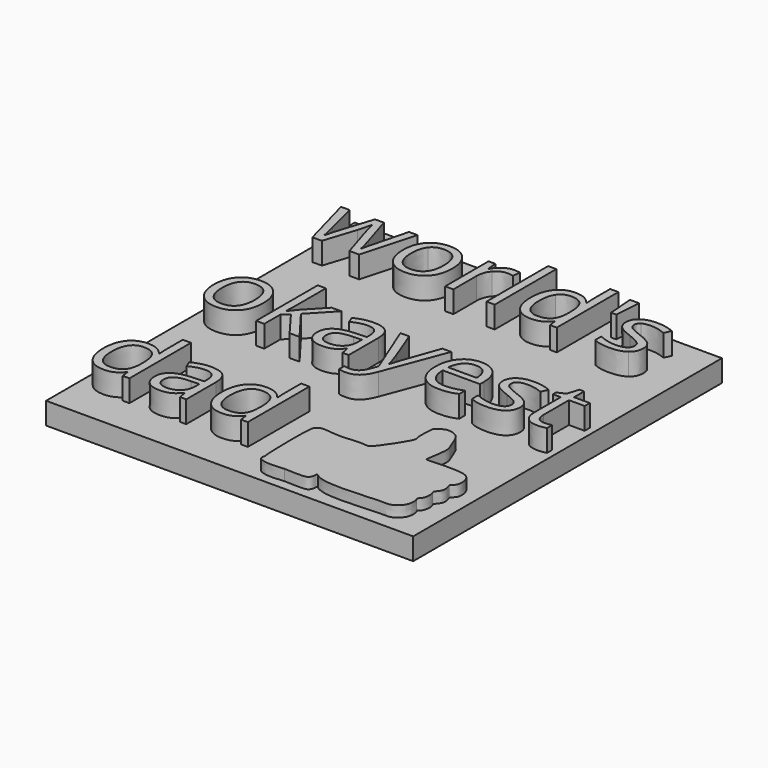
from build123d import *

# Parameters (mm, degrees)
F0_W         = 0.954216132
F0_H         = 0.4688345157
F0_H_2       = 8.4721154837
F1_DEPTH     = 5.08
F0_TEXT_SIZE = 11.7668270607
F2_DEPTH     = 5.08
F3_DEPTH     = 5.08
F4_DEPTH     = 2.54
F6_DEPTH     = 1.27


# Not quite as in the source:
# - Text() gives the source's letters only with a copy of the font that has no kerning and outlines rounded to 1/6400 em; it was checked with that copy


with BuildPart() as f1:
    # F0 (on Top) → F1 (new body)
    with BuildSketch(Plane.XY):
        with Locations((1.2318397079, 22.6472947877)):
            Rectangle(F0_W, F0_H)
        with Locations((8.4426984161, 22.6472947877)):
            Rectangle(F0_W, F0_H)
        with Locations((1.2318397079, 18.176819788)):
            Rectangle(F0_W, F0_H_2)
        with BuildLine():
            Line((8.9198064821, 22.4128775299), (7.9655903501, 22.4128775299))
            Line((7.9655903501, 22.4128775299), (7.9655903501, 20.3187500264))
            Line((7.9655903501, 20.3187500264), (7.9894917176, 19.8756554449))
            Line((7.9894917176, 19.8756554449), (8.0299401856, 19.421529463))
            Line((8.0299401856, 19.421529463), (7.9545589497, 19.421529463))
            add(Edge.make_bspline(
                [(5.9891311172, 20.3536827942), (7.2706121268, 20.3536827942), (7.9545589497, 19.421529463)],
                knots=[0, 0, 0, 1, 1, 1], degree=2))
            add(Edge.make_bspline(
                [(4.069667453, 19.4913949987), (4.759129976, 20.3536827942), (5.9891311172, 20.3536827942)],
                knots=[0, 0, 0, 1, 1, 1], degree=2))
            add(Edge.make_bspline(
                [(3.3802049299, 17.0718411843), (3.3802049299, 18.6291072031), (4.069667453, 19.4913949987)],
                knots=[0, 0, 0, 1, 1, 1], degree=2))
            add(Edge.make_bspline(
                [(4.0669096029, 14.6697537539), (3.3802049299, 15.5145751655), (3.3802049299, 17.0718411843)],
                knots=[0, 0, 0, 1, 1, 1], degree=2))
            add(Edge.make_bspline(
                [(5.9891311172, 13.8249323423), (4.7536142759, 13.8249323423), (4.0669096029, 14.6697537539)],
                knots=[0, 0, 0, 1, 1, 1], degree=2))
            add(Edge.make_bspline(
                [(7.9655903501, 14.7846641744), (7.3055448947, 13.8249323423), (5.9891311172, 13.8249323423)],
                knots=[0, 0, 0, 1, 1, 1], degree=2))
            Line((7.9655903501, 14.7846641744), (8.0170702185, 14.7846641744))
            Line((8.0170702185, 14.7846641744), (8.1439313227, 13.9407620461))
            Line((8.1439313227, 13.9407620461), (8.9198064821, 13.9407620461))
            Line((8.9198064821, 13.9407620461), (8.9198064821, 22.4128775299))
        make_face()
        with BuildLine():
            add(Edge.make_bspline(
                [(6.1104765213, 14.624708869), (7.086755454, 14.624708869), (7.526172902, 15.1560546535)],
                knots=[0, 0, 0, 1, 1, 1], degree=2))
            add(Edge.make_bspline(
                [(4.8115291278, 15.2397094396), (5.2537044259, 14.624708869), (6.1104765213, 14.624708869)],
                knots=[0, 0, 0, 1, 1, 1], degree=2))
            add(Edge.make_bspline(
                [(4.3693538297, 17.060809784), (4.3693538297, 15.8547100102), (4.8115291278, 15.2397094396)],
                knots=[0, 0, 0, 1, 1, 1], degree=2))
            add(Edge.make_bspline(
                [(4.8142869779, 18.9021343623), (4.3693538297, 18.2503624571), (4.3693538297, 17.060809784)],
                knots=[0, 0, 0, 1, 1, 1], degree=2))
            add(Edge.make_bspline(
                [(6.0994451209, 19.5539062674), (5.2592201261, 19.5539062674), (4.8142869779, 18.9021343623)],
                knots=[0, 0, 0, 1, 1, 1], degree=2))
            add(Edge.make_bspline(
                [(7.5206572019, 18.982112015), (7.0757240536, 19.5539062674), (6.0994451209, 19.5539062674)],
                knots=[0, 0, 0, 1, 1, 1], degree=2))
            add(Edge.make_bspline(
                [(7.9655903501, 17.0718411843), (7.9655903501, 18.4103177625), (7.5206572019, 18.982112015)],
                knots=[0, 0, 0, 1, 1, 1], degree=2))
            Line((7.9655903501, 17.0718411843), (7.9655903501, 16.8714374109))
            add(Edge.make_bspline(
                [(7.526172902, 15.1560546535), (7.9655903501, 15.687400438), (7.9655903501, 16.8714374109)],
                knots=[0, 0, 0, 1, 1, 1], degree=2))
        make_face(mode=Mode.SUBTRACT)
        with BuildLine():
            add(Edge.make_bspline(
                [(-1.1757634227, 20.3536827942), (-0.7565702087, 20.3536827942), (-0.4237896309, 20.2838172586)],
                knots=[0, 0, 0, 1, 1, 1], degree=2))
            add(Edge.make_bspline(
                [(-2.2623563591, 20.0199829331), (-1.7677819092, 20.3536827942), (-1.1757634227, 20.3536827942)],
                knots=[0, 0, 0, 1, 1, 1], degree=2))
            add(Edge.make_bspline(
                [(-3.1062584874, 19.0722017846), (-2.756930809, 19.6862830719), (-2.2623563591, 20.0199829331)],
                knots=[0, 0, 0, 1, 1, 1], degree=2))
            Line((-3.1062584874, 19.0722017846), (-3.1522226556, 19.0722017846))
            Line((-3.1522226556, 19.0722017846), (-3.2625366593, 20.2378530904))
            Line((-3.2625366593, 20.2378530904), (-4.0494432189, 20.2378530904))
            Line((-4.0494432189, 20.2378530904), (-4.0494432189, 13.9407620461))
            Line((-4.0494432189, 13.9407620461), (-3.095227087, 13.9407620461))
            Line((-3.095227087, 13.9407620461), (-3.095227087, 17.3200476926))
            add(Edge.make_bspline(
                [(-2.5528499022, 18.8653630277), (-3.095227087, 18.2448467569), (-3.095227087, 17.3200476926)],
                knots=[0, 0, 0, 1, 1, 1], degree=2))
            add(Edge.make_bspline(
                [(-1.2456289584, 19.4858792985), (-2.0104727173, 19.4858792985), (-2.5528499022, 18.8653630277)],
                knots=[0, 0, 0, 1, 1, 1], degree=2))
            add(Edge.make_bspline(
                [(-0.5561664353, 19.3994666623), (-0.9459425817, 19.4858792985), (-1.2456289584, 19.4858792985)],
                knots=[0, 0, 0, 1, 1, 1], degree=2))
            Line((-0.5561664353, 19.3994666623), (-0.4237896309, 20.2838172586))
        make_face()
        with BuildLine():
            add(Edge.make_bspline(
                [(-5.7225389416, 17.0957425518), (-5.7225389416, 15.5550236335), (-6.4974948176, 14.6899779879)],
                knots=[0, 0, 0, 1, 1, 1], degree=2))
            add(Edge.make_bspline(
                [(-6.5011719511, 19.4739286148), (-5.7225389416, 18.5941744353), (-5.7225389416, 17.0957425518)],
                knots=[0, 0, 0, 1, 1, 1], degree=2))
            add(Edge.make_bspline(
                [(-8.5998958713, 20.3536827942), (-7.2798049605, 20.3536827942), (-6.5011719511, 19.4739286148)],
                knots=[0, 0, 0, 1, 1, 1], degree=2))
            add(Edge.make_bspline(
                [(-10.7381489763, 19.4941528488), (-9.9677895171, 20.3536827942), (-8.5998958713, 20.3536827942)],
                knots=[0, 0, 0, 1, 1, 1], degree=2))
            add(Edge.make_bspline(
                [(-11.5085084354, 17.0957425518), (-11.5085084354, 18.6346229033), (-10.7381489763, 19.4941528488)],
                knots=[0, 0, 0, 1, 1, 1], degree=2))
            add(Edge.make_bspline(
                [(-11.1518264901, 15.3601355603), (-11.5085084354, 16.1010779518), (-11.5085084354, 17.0957425518)],
                knots=[0, 0, 0, 1, 1, 1], degree=2))
            add(Edge.make_bspline(
                [(-10.1406147896, 14.2220627556), (-10.7951445449, 14.6191931689), (-11.1518264901, 15.3601355603)],
                knots=[0, 0, 0, 1, 1, 1], degree=2))
            add(Edge.make_bspline(
                [(-8.6403443394, 13.8249323423), (-9.4860850344, 13.8249323423), (-10.1406147896, 14.2220627556)],
                knots=[0, 0, 0, 1, 1, 1], degree=2))
            add(Edge.make_bspline(
                [(-6.4974948176, 14.6899779879), (-7.2724506936, 13.8249323423), (-8.6403443394, 13.8249323423)],
                knots=[0, 0, 0, 1, 1, 1], degree=2))
        make_face()
        with BuildLine():
            add(Edge.make_bspline(
                [(-10.5193595356, 17.0957425518), (-10.5193595356, 15.8878042113), (-10.0367357695, 15.2562565402)],
                knots=[0, 0, 0, 1, 1, 1], degree=2))
            add(Edge.make_bspline(
                [(-10.0422514696, 18.9278742965), (-10.5193595356, 18.3128737259), (-10.5193595356, 17.0957425518)],
                knots=[0, 0, 0, 1, 1, 1], degree=2))
            add(Edge.make_bspline(
                [(-8.629312939, 19.5428748671), (-9.5651434037, 19.5428748671), (-10.0422514696, 18.9278742965)],
                knots=[0, 0, 0, 1, 1, 1], degree=2))
            add(Edge.make_bspline(
                [(-7.195230891, 18.9196007462), (-7.6806125072, 19.5428748671), (-8.629312939, 19.5428748671)],
                knots=[0, 0, 0, 1, 1, 1], degree=2))
            add(Edge.make_bspline(
                [(-6.7098492747, 17.0957425518), (-6.7098492747, 18.2963266253), (-7.195230891, 18.9196007462)],
                knots=[0, 0, 0, 1, 1, 1], degree=2))
            add(Edge.make_bspline(
                [(-7.195230891, 15.2534986901), (-6.7098492747, 15.8822885112), (-6.7098492747, 17.0957425518)],
                knots=[0, 0, 0, 1, 1, 1], degree=2))
            add(Edge.make_bspline(
                [(-8.6182815386, 14.624708869), (-7.6806125072, 14.624708869), (-7.195230891, 15.2534986901)],
                knots=[0, 0, 0, 1, 1, 1], degree=2))
            add(Edge.make_bspline(
                [(-10.0367357695, 15.2562565402), (-9.5541120033, 14.624708869), (-8.6182815386, 14.624708869)],
                knots=[0, 0, 0, 1, 1, 1], degree=2))
        make_face(mode=Mode.SUBTRACT)
        with BuildLine():
            Line((-16.3218761299, 17.6344426032), (-15.1672562246, 13.9407620461))
            Line((-15.1672562246, 13.9407620461), (-14.03469912, 13.9407620461))
            Line((-14.03469912, 13.9407620461), (-12.2954149951, 20.2378530904))
            Line((-12.2954149951, 20.2378530904), (-13.2827253282, 20.2378530904))
            add(Edge.make_bspline(
                [(-14.4805515516, 15.6019070851), (-14.3803496649, 16.0330509829), (-13.2827253282, 20.2378530904)],
                knots=[0, 0, 0, 1, 1, 1], degree=2))
            add(Edge.make_bspline(
                [(-14.6046548058, 14.963005147), (-14.5807534383, 15.1707631873), (-14.4805515516, 15.6019070851)],
                knots=[0, 0, 0, 1, 1, 1], degree=2))
            Line((-14.6046548058, 14.963005147), (-14.650618974, 14.963005147))
            add(Edge.make_bspline(
                [(-15.0863592886, 16.6232309026), (-14.7646101111, 15.6359205696), (-14.650618974, 14.963005147)],
                knots=[0, 0, 0, 1, 1, 1], degree=2))
            Line((-15.0863592886, 16.6232309026), (-16.213400693, 20.2378530904))
            Line((-16.213400693, 20.2378530904), (-17.2466751942, 20.2378530904))
            Line((-17.2466751942, 20.2378530904), (-18.4012950996, 16.6232309026))
            add(Edge.make_bspline(
                [(-18.6467437578, 15.7995530084), (-18.5060934031, 16.3198673925), (-18.4012950996, 16.6232309026)],
                knots=[0, 0, 0, 1, 1, 1], degree=2))
            add(Edge.make_bspline(
                [(-18.8499053813, 14.9519737467), (-18.7873941125, 15.2792386243), (-18.6467437578, 15.7995530084)],
                knots=[0, 0, 0, 1, 1, 1], degree=2))
            Line((-18.8499053813, 14.9519737467), (-18.8958695495, 14.9519737467))
            add(Edge.make_bspline(
                [(-19.260825045, 16.6232309026), (-18.9418337177, 15.3821983611), (-18.8958695495, 14.9519737467)],
                knots=[0, 0, 0, 1, 1, 1], degree=2))
            add(Edge.make_bspline(
                [(-20.1883819594, 20.2378530904), (-19.5798163724, 17.8642634442), (-19.260825045, 16.6232309026)],
                knots=[0, 0, 0, 1, 1, 1], degree=2))
            Line((-20.1883819594, 20.2378530904), (-21.1885622596, 20.2378530904))
            Line((-21.1885622596, 20.2378530904), (-19.4713409354, 13.9407620461))
            Line((-19.4713409354, 13.9407620461), (-18.3682008985, 13.9407620461))
            Line((-18.3682008985, 13.9407620461), (-17.1786482253, 17.6234112028))
            add(Edge.make_bspline(
                [(-16.7760021118, 19.1751615214), (-17.0058229528, 18.1694655211), (-17.1786482253, 17.6234112028)],
                knots=[0, 0, 0, 1, 1, 1], degree=2))
            Line((-16.7760021118, 19.1751615214), (-16.7300379436, 19.1751615214))
            add(Edge.make_bspline(
                [(-16.3218761299, 17.6344426032), (-16.4321901336, 17.9745774479), (-16.7300379436, 19.1751615214)],
                knots=[0, 0, 0, 1, 1, 1], degree=2))
        make_face()
        Polygon((11.5342483696, 19.3075383259), (11.7640692106, 22.3411734275), (10.6958619415, 22.3411734275), (10.9311984827, 19.3075383259), align=None)
        with BuildLine():
            add(Edge.make_bspline(
                [(17.607034273, 15.6579833703), (17.607034273, 14.7791484742), (16.9525045177, 14.3020404082)],
                knots=[0, 0, 0, 1, 1, 1], degree=2))
            add(Edge.make_bspline(
                [(17.2135809931, 16.6986121385), (17.607034273, 16.2849346246), (17.607034273, 15.6579833703)],
                knots=[0, 0, 0, 1, 1, 1], degree=2))
            add(Edge.make_bspline(
                [(15.7004405758, 17.520451466), (16.8201277133, 17.1122896523), (17.2135809931, 16.6986121385)],
                knots=[0, 0, 0, 1, 1, 1], degree=2))
            add(Edge.make_bspline(
                [(14.5973005389, 17.9865281316), (14.8841169485, 17.8256535429), (15.7004405758, 17.520451466)],
                knots=[0, 0, 0, 1, 1, 1], degree=2))
            add(Edge.make_bspline(
                [(14.1808651749, 18.3248244096), (14.3104841292, 18.1474027203), (14.5973005389, 17.9865281316)],
                knots=[0, 0, 0, 1, 1, 1], degree=2))
            add(Edge.make_bspline(
                [(14.0512462206, 18.7559683074), (14.0512462206, 18.5022460989), (14.1808651749, 18.3248244096)],
                knots=[0, 0, 0, 1, 1, 1], degree=2))
            add(Edge.make_bspline(
                [(14.3959774821, 19.3415518103), (14.0512462206, 19.1291973532), (14.0512462206, 18.7559683074)],
                knots=[0, 0, 0, 1, 1, 1], degree=2))
            add(Edge.make_bspline(
                [(15.4191398664, 19.5539062674), (14.7407087437, 19.5539062674), (14.3959774821, 19.3415518103)],
                knots=[0, 0, 0, 1, 1, 1], degree=2))
            add(Edge.make_bspline(
                [(17.1363611906, 19.1641301211), (16.1894993255, 19.5539062674), (15.4191398664, 19.5539062674)],
                knots=[0, 0, 0, 1, 1, 1], degree=2))
            Line((17.1363611906, 19.1641301211), (17.4764960353, 19.9400052804))
            add(Edge.make_bspline(
                [(15.4871668353, 20.3536827942), (16.503894236, 20.3536827942), (17.4764960353, 19.9400052804)],
                knots=[0, 0, 0, 1, 1, 1], degree=2))
            add(Edge.make_bspline(
                [(13.7699455111, 19.9078303626), (14.3968967655, 20.3536827942), (15.4871668353, 20.3536827942)],
                knots=[0, 0, 0, 1, 1, 1], degree=2))
            add(Edge.make_bspline(
                [(13.1429942568, 18.6916184719), (13.1429942568, 19.461977931), (13.7699455111, 19.9078303626)],
                knots=[0, 0, 0, 1, 1, 1], degree=2))
            add(Edge.make_bspline(
                [(13.3240930795, 17.9515953638), (13.1429942568, 18.2613938575), (13.1429942568, 18.6916184719)],
                knots=[0, 0, 0, 1, 1, 1], degree=2))
            add(Edge.make_bspline(
                [(13.875663098, 17.3972674952), (13.5051919023, 17.6417968701), (13.3240930795, 17.9515953638)],
                knots=[0, 0, 0, 1, 1, 1], degree=2))
            add(Edge.make_bspline(
                [(15.1249691899, 16.8254732427), (14.2461342938, 17.1527381204), (13.875663098, 17.3972674952)],
                knots=[0, 0, 0, 1, 1, 1], degree=2))
            add(Edge.make_bspline(
                [(16.3696788649, 16.2077148221), (16.0516068209, 16.4687912975), (15.1249691899, 16.8254732427)],
                knots=[0, 0, 0, 1, 1, 1], degree=2))
            add(Edge.make_bspline(
                [(16.6877509089, 15.578925001), (16.6877509089, 15.9466383466), (16.3696788649, 16.2077148221)],
                knots=[0, 0, 0, 1, 1, 1], degree=2))
            add(Edge.make_bspline(
                [(16.2860240787, 14.85177186), (16.6877509089, 15.0898662513), (16.6877509089, 15.578925001)],
                knots=[0, 0, 0, 1, 1, 1], degree=2))
            add(Edge.make_bspline(
                [(15.137839157, 14.6136774687), (15.8842972486, 14.6136774687), (16.2860240787, 14.85177186)],
                knots=[0, 0, 0, 1, 1, 1], degree=2))
            add(Edge.make_bspline(
                [(14.1349010067, 14.7451349897), (14.6542961074, 14.6136774687), (15.137839157, 14.6136774687)],
                knots=[0, 0, 0, 1, 1, 1], degree=2))
            add(Edge.make_bspline(
                [(13.1613799241, 15.1064133518), (13.615505906, 14.8765925108), (14.1349010067, 14.7451349897)],
                knots=[0, 0, 0, 1, 1, 1], degree=2))
            Line((13.1613799241, 15.1064133518), (13.1613799241, 14.2220627556))
            add(Edge.make_bspline(
                [(15.1139377895, 13.8249323423), (13.8618738476, 13.8249323423), (13.1613799241, 14.2220627556)],
                knots=[0, 0, 0, 1, 1, 1], degree=2))
            add(Edge.make_bspline(
                [(16.9525045177, 14.3020404082), (16.2979747625, 13.8249323423), (15.1139377895, 13.8249323423)],
                knots=[0, 0, 0, 1, 1, 1], degree=2))
        make_face()
    extrude(amount=F1_DEPTH)



with BuildPart() as f2:
    # F0 (on Top) → F2 (new body)
    with BuildSketch(Plane.XY):
        with Locations((-21.320939064, -2.0621227565)):
            Text('okayest', F0_TEXT_SIZE, font='Open Sans', text_align=(TextAlign.LEFT, TextAlign.BOTTOM))
    extrude(amount=F2_DEPTH)


with BuildPart() as f3:
    # F0 (on Top) → F3 (new body)
    with BuildSketch(Plane.XY):
        with Locations((-21.320939064, -18.0650075591)):
            Text('dad', F0_TEXT_SIZE, font='Open Sans', text_align=(TextAlign.LEFT, TextAlign.BOTTOM))
    extrude(amount=F3_DEPTH)


with BuildPart() as f1_1:
    add(f1.part)

    add(f2.part)  # F4 merges F2

    add(f3.part)  # F4 merges F3
    # F0 (on Top) → F4 (join)
    with BuildSketch(Plane.XY):
        with BuildLine():
            Line((0.7547316419, 22.4128775299), (-21.320939064, 22.4128775299))
            Line((-21.320939064, 22.4128775299), (-21.320939064, -22.4128775299))
            Line((-21.320939064, -22.4128775299), (21.320939064, -22.4128775299))
            Line((21.320939064, -22.4128775299), (21.320939064, 22.4128775299))
            Line((21.320939064, 22.4128775299), (8.9198064821, 22.4128775299))
            Line((8.9198064821, 22.4128775299), (8.9198064821, 13.9407620461))
            Line((8.9198064821, 13.9407620461), (8.1439313227, 13.9407620461))
            Line((8.1439313227, 13.9407620461), (8.0170702185, 14.7846641744))
            Line((8.0170702185, 14.7846641744), (7.9655903501, 14.7846641744))
            add(Edge.make_bspline(
                [(7.9655903501, 14.7846641744), (7.3055448947, 13.8249323423), (5.9891311172, 13.8249323423)],
                knots=[0, 0, 0, 1, 1, 1], degree=2))
            add(Edge.make_bspline(
                [(5.9891311172, 13.8249323423), (4.7536142759, 13.8249323423), (4.0669096029, 14.6697537539)],
                knots=[0, 0, 0, 1, 1, 1], degree=2))
            add(Edge.make_bspline(
                [(4.0669096029, 14.6697537539), (3.3802049299, 15.5145751655), (3.3802049299, 17.0718411843)],
                knots=[0, 0, 0, 1, 1, 1], degree=2))
            add(Edge.make_bspline(
                [(3.3802049299, 17.0718411843), (3.3802049299, 18.6291072031), (4.069667453, 19.4913949987)],
                knots=[0, 0, 0, 1, 1, 1], degree=2))
            add(Edge.make_bspline(
                [(4.069667453, 19.4913949987), (4.759129976, 20.3536827942), (5.9891311172, 20.3536827942)],
                knots=[0, 0, 0, 1, 1, 1], degree=2))
            add(Edge.make_bspline(
                [(5.9891311172, 20.3536827942), (7.2706121268, 20.3536827942), (7.9545589497, 19.421529463)],
                knots=[0, 0, 0, 1, 1, 1], degree=2))
            Line((7.9545589497, 19.421529463), (8.0299401856, 19.421529463))
            Line((8.0299401856, 19.421529463), (7.9894917176, 19.8756554449))
            Line((7.9894917176, 19.8756554449), (7.9655903501, 20.3187500264))
            Line((7.9655903501, 20.3187500264), (7.9655903501, 22.4128775299))
            Line((7.9655903501, 22.4128775299), (1.7089477739, 22.4128775299))
            Line((1.7089477739, 22.4128775299), (1.7089477739, 13.9407620461))
            Line((1.7089477739, 13.9407620461), (0.7547316419, 13.9407620461))
            Line((0.7547316419, 13.9407620461), (0.7547316419, 22.4128775299))
        make_face()
        with BuildLine():
            Line((-15.8971672157, -18.0650075591), (-16.02402832, -17.2211054308))
            Line((-16.02402832, -17.2211054308), (-16.0755081884, -17.2211054308))
            add(Edge.make_bspline(
                [(-16.0755081884, -17.2211054308), (-16.7355536438, -18.1808372629), (-18.0519674212, -18.1808372629)],
                knots=[0, 0, 0, 1, 1, 1], degree=2))
            add(Edge.make_bspline(
                [(-18.0519674212, -18.1808372629), (-19.2874842626, -18.1808372629), (-19.9741889356, -17.3360158513)],
                knots=[0, 0, 0, 1, 1, 1], degree=2))
            add(Edge.make_bspline(
                [(-19.9741889356, -17.3360158513), (-20.6608936086, -16.4911944397), (-20.6608936086, -14.9339284209)],
                knots=[0, 0, 0, 1, 1, 1], degree=2))
            add(Edge.make_bspline(
                [(-20.6608936086, -14.9339284209), (-20.6608936086, -13.376662402), (-19.9714310855, -12.5143746065)],
                knots=[0, 0, 0, 1, 1, 1], degree=2))
            add(Edge.make_bspline(
                [(-19.9714310855, -12.5143746065), (-19.2819685624, -11.652086811), (-18.0519674212, -11.652086811)],
                knots=[0, 0, 0, 1, 1, 1], degree=2))
            add(Edge.make_bspline(
                [(-18.0519674212, -11.652086811), (-16.7704864116, -11.652086811), (-16.0865395887, -12.5842401422)],
                knots=[0, 0, 0, 1, 1, 1], degree=2))
            Line((-16.0865395887, -12.5842401422), (-16.0111583529, -12.5842401422))
            Line((-16.0111583529, -12.5842401422), (-16.0516068209, -12.1301141603))
            Line((-16.0516068209, -12.1301141603), (-16.0755081884, -11.6870195788))
            Line((-16.0755081884, -11.6870195788), (-16.0755081884, -9.1240575596))
            Line((-16.0755081884, -9.1240575596), (-15.1212920564, -9.1240575596))
            Line((-15.1212920564, -9.1240575596), (-15.1212920564, -18.0650075591))
            Line((-15.1212920564, -18.0650075591), (-15.8971672157, -18.0650075591))
        make_face(mode=Mode.SUBTRACT)
        with BuildLine():
            Line((-8.5189989353, -18.0650075591), (-9.2268471257, -18.0650075591))
            Line((-9.2268471257, -18.0650075591), (-9.4162194987, -17.1677869957))
            Line((-9.4162194987, -17.1677869957), (-9.4621836669, -17.1677869957))
            add(Edge.make_bspline(
                [(-9.4621836669, -17.1677869957), (-9.9328567493, -17.7598054822), (-10.4007719816, -17.9703213726)],
                knots=[0, 0, 0, 1, 1, 1], degree=2))
            add(Edge.make_bspline(
                [(-10.4007719816, -17.9703213726), (-10.868687214, -18.1808372629), (-11.5710197042, -18.1808372629)],
                knots=[0, 0, 0, 1, 1, 1], degree=2))
            add(Edge.make_bspline(
                [(-11.5710197042, -18.1808372629), (-12.5068501688, -18.1808372629), (-13.0381959533, -17.6972942134)],
                knots=[0, 0, 0, 1, 1, 1], degree=2))
            add(Edge.make_bspline(
                [(-13.0381959533, -17.6972942134), (-13.5695417378, -17.2137511639), (-13.5695417378, -16.3238848674)],
                knots=[0, 0, 0, 1, 1, 1], degree=2))
            add(Edge.make_bspline(
                [(-13.5695417378, -16.3238848674), (-13.5695417378, -14.4172911702), (-10.5193595356, -14.3253628338)],
                knots=[0, 0, 0, 1, 1, 1], degree=2))
            Line((-10.5193595356, -14.3253628338), (-9.4511522665, -14.290430066))
            Line((-9.4511522665, -14.290430066), (-9.4511522665, -13.8988153529))
            add(Edge.make_bspline(
                [(-9.4511522665, -13.8988153529), (-9.4511522665, -13.1578729614), (-9.7692243105, -12.8048681496)],
                knots=[0, 0, 0, 1, 1, 1], degree=2))
            add(Edge.make_bspline(
                [(-9.7692243105, -12.8048681496), (-10.0872963545, -12.4518633377), (-10.7896288447, -12.4518633377)],
                knots=[0, 0, 0, 1, 1, 1], degree=2))
            add(Edge.make_bspline(
                [(-10.7896288447, -12.4518633377), (-11.5765354044, -12.4518633377), (-12.5693614376, -12.9335678205)],
                knots=[0, 0, 0, 1, 1, 1], degree=2))
            Line((-12.5693614376, -12.9335678205), (-12.8635321141, -12.2036568294))
            add(Edge.make_bspline(
                [(-12.8635321141, -12.2036568294), (-12.3983747319, -11.9517731877), (-11.8440468633, -11.8083649829)],
                knots=[0, 0, 0, 1, 1, 1], degree=2))
            add(Edge.make_bspline(
                [(-11.8440468633, -11.8083649829), (-11.2897189948, -11.6649567781), (-10.7307947094, -11.6649567781)],
                knots=[0, 0, 0, 1, 1, 1], degree=2))
            add(Edge.make_bspline(
                [(-10.7307947094, -11.6649567781), (-9.6055918717, -11.6649567781), (-9.0622954035, -12.1641276448)],
                knots=[0, 0, 0, 1, 1, 1], degree=2))
            add(Edge.make_bspline(
                [(-9.0622954035, -12.1641276448), (-8.5189989353, -12.6632985115), (-8.5189989353, -13.7664385484)],
                knots=[0, 0, 0, 1, 1, 1], degree=2))
            Line((-8.5189989353, -13.7664385484), (-8.5189989353, -18.0650075591))
        make_face(mode=Mode.SUBTRACT)
        with BuildLine():
            Line((-2.1428495218, -18.0650075591), (-2.269710626, -17.2211054308))
            Line((-2.269710626, -17.2211054308), (-2.3211904944, -17.2211054308))
            add(Edge.make_bspline(
                [(-2.3211904944, -17.2211054308), (-2.9812359498, -18.1808372629), (-4.2976497273, -18.1808372629)],
                knots=[0, 0, 0, 1, 1, 1], degree=2))
            add(Edge.make_bspline(
                [(-4.2976497273, -18.1808372629), (-5.5331665686, -18.1808372629), (-6.2198712416, -17.3360158513)],
                knots=[0, 0, 0, 1, 1, 1], degree=2))
            add(Edge.make_bspline(
                [(-6.2198712416, -17.3360158513), (-6.9065759146, -16.4911944397), (-6.9065759146, -14.9339284209)],
                knots=[0, 0, 0, 1, 1, 1], degree=2))
            add(Edge.make_bspline(
                [(-6.9065759146, -14.9339284209), (-6.9065759146, -13.376662402), (-6.2171133915, -12.5143746065)],
                knots=[0, 0, 0, 1, 1, 1], degree=2))
            add(Edge.make_bspline(
                [(-6.2171133915, -12.5143746065), (-5.5276508685, -11.652086811), (-4.2976497273, -11.652086811)],
                knots=[0, 0, 0, 1, 1, 1], degree=2))
            add(Edge.make_bspline(
                [(-4.2976497273, -11.652086811), (-3.0161687177, -11.652086811), (-2.3322218948, -12.5842401422)],
                knots=[0, 0, 0, 1, 1, 1], degree=2))
            Line((-2.3322218948, -12.5842401422), (-2.2568406589, -12.5842401422))
            Line((-2.2568406589, -12.5842401422), (-2.2972891269, -12.1301141603))
            Line((-2.2972891269, -12.1301141603), (-2.3211904944, -11.6870195788))
            Line((-2.3211904944, -11.6870195788), (-2.3211904944, -9.1240575596))
            Line((-2.3211904944, -9.1240575596), (-1.3669743624, -9.1240575596))
            Line((-1.3669743624, -9.1240575596), (-1.3669743624, -18.0650075591))
            Line((-1.3669743624, -18.0650075591), (-2.1428495218, -18.0650075591))
        make_face(mode=Mode.SUBTRACT)
        with BuildLine():
            Line((1.0580951521, -2.0970555243), (-1.4828040663, 4.2349682878))
            Line((-1.4828040663, 4.2349682878), (-0.4587223987, 4.2349682878))
            Line((-0.4587223987, 4.2349682878), (0.9202026475, 0.6442474675))
            add(Edge.make_bspline(
                [(0.9202026475, 0.6442474675), (1.3724900626, -0.5857536737), (1.4828040663, -1.131807992)],
                knots=[0, 0, 0, 1, 1, 1], degree=2))
            Line((1.4828040663, -1.131807992), (1.5287682345, -1.131807992))
            add(Edge.make_bspline(
                [(1.5287682345, -1.131807992), (1.6023109037, -0.8376373155), (1.8413245783, -0.1279505584)],
                knots=[0, 0, 0, 1, 1, 1], degree=2))
            add(Edge.make_bspline(
                [(1.8413245783, -0.1279505584), (2.080338253, 0.5817361987), (3.4022677306, 4.2349682878)],
                knots=[0, 0, 0, 1, 1, 1], degree=2))
            Line((3.4022677306, 4.2349682878), (4.4245108315, 4.2349682878))
            Line((4.4245108315, 4.2349682878), (1.7181406075, -2.9354419524))
            add(Edge.make_bspline(
                [(1.7181406075, -2.9354419524), (1.3154944941, -3.9981335213), (0.7786330094, -4.4439859529)],
                knots=[0, 0, 0, 1, 1, 1], degree=2))
            add(Edge.make_bspline(
                [(0.7786330094, -4.4439859529), (0.2417715248, -4.8898383845), (-0.5396193347, -4.8898383845)],
                knots=[0, 0, 0, 1, 1, 1], degree=2))
            add(Edge.make_bspline(
                [(-0.5396193347, -4.8898383845), (-0.9771982161, -4.8898383845), (-1.4019071303, -4.7905557812)],
                knots=[0, 0, 0, 1, 1, 1], degree=2))
            Line((-1.4019071303, -4.7905557812), (-1.4019071303, -4.0275505889))
            add(Edge.make_bspline(
                [(-1.4019071303, -4.0275505889), (-1.085673653, -4.0955775579), (-0.6958975066, -4.0955775579)],
                knots=[0, 0, 0, 1, 1, 1], degree=2))
            add(Edge.make_bspline(
                [(-0.6958975066, -4.0955775579), (0.287735693, -4.0955775579), (0.706928907, -2.9924375209)],
                knots=[0, 0, 0, 1, 1, 1], degree=2))
            Line((0.706928907, -2.9924375209), (1.0580951521, -2.0970555243))
        make_face(mode=Mode.SUBTRACT)
        with BuildLine():
            add(Edge.make_bspline(
                [(-15.6535571242, 3.4710438122), (-14.8749241148, 2.5912896327), (-14.8749241148, 1.0928577492)],
                knots=[0, 0, 0, 1, 1, 1], degree=2))
            add(Edge.make_bspline(
                [(-14.8749241148, 1.0928577492), (-14.8749241148, -0.4478611691), (-15.6498799908, -1.3129068147)],
                knots=[0, 0, 0, 1, 1, 1], degree=2))
            add(Edge.make_bspline(
                [(-15.6498799908, -1.3129068147), (-16.4248358667, -2.1779524603), (-17.7927295125, -2.1779524603)],
                knots=[0, 0, 0, 1, 1, 1], degree=2))
            add(Edge.make_bspline(
                [(-17.7927295125, -2.1779524603), (-18.6384702075, -2.1779524603), (-19.2929999628, -1.780822047)],
                knots=[0, 0, 0, 1, 1, 1], degree=2))
            add(Edge.make_bspline(
                [(-19.2929999628, -1.780822047), (-19.947529718, -1.3836916337), (-20.3042116633, -0.6427492423)],
                knots=[0, 0, 0, 1, 1, 1], degree=2))
            add(Edge.make_bspline(
                [(-20.3042116633, -0.6427492423), (-20.6608936086, 0.0981931492), (-20.6608936086, 1.0928577492)],
                knots=[0, 0, 0, 1, 1, 1], degree=2))
            add(Edge.make_bspline(
                [(-20.6608936086, 1.0928577492), (-20.6608936086, 2.6317381007), (-19.8905341495, 3.4912680462)],
                knots=[0, 0, 0, 1, 1, 1], degree=2))
            add(Edge.make_bspline(
                [(-19.8905341495, 3.4912680462), (-19.1201746903, 4.3507979916), (-17.7522810445, 4.3507979916)],
                knots=[0, 0, 0, 1, 1, 1], degree=2))
            add(Edge.make_bspline(
                [(-17.7522810445, 4.3507979916), (-16.4321901336, 4.3507979916), (-15.6535571242, 3.4710438122)],
                knots=[0, 0, 0, 1, 1, 1], degree=2))
        make_face(mode=Mode.SUBTRACT)
        with BuildLine():
            Line((-12.3046078287, 1.1608847181), (-12.2586436605, 1.1608847181))
            add(Edge.make_bspline(
                [(-12.2586436605, 1.1608847181), (-12.012275719, 1.5120509632), (-11.5066698687, 2.0801680823)],
                knots=[0, 0, 0, 1, 1, 1], degree=2))
            Line((-11.5066698687, 2.0801680823), (-9.4732150673, 4.2349682878))
            Line((-9.4732150673, 4.2349682878), (-8.3406579627, 4.2349682878))
            Line((-8.3406579627, 4.2349682878), (-10.8925885815, 1.5524994313))
            Line((-10.8925885815, 1.5524994313), (-8.16231699, -2.0621227565))
            Line((-8.16231699, -2.0621227565), (-9.3169368954, -2.0621227565))
            Line((-9.3169368954, -2.0621227565), (-11.5416026365, 0.9145167766))
            Line((-11.5416026365, 0.9145167766), (-12.2586436605, 0.2930812224))
            Line((-12.2586436605, 0.2930812224), (-12.2586436605, -2.0621227565))
            Line((-12.2586436605, -2.0621227565), (-13.2018283921, -2.0621227565))
            Line((-13.2018283921, -2.0621227565), (-13.2018283921, 6.878827243))
            Line((-13.2018283921, 6.878827243), (-12.2586436605, 6.878827243))
            Line((-12.2586436605, 6.878827243), (-12.2586436605, 2.1371636508))
            add(Edge.make_bspline(
                [(-12.2586436605, 2.1371636508), (-12.2586436605, 1.8227687403), (-12.3046078287, 1.1608847181)],
                knots=[0, 0, 0, 1, 1, 1], degree=2))
        make_face(mode=Mode.SUBTRACT)
        with BuildLine():
            Line((-2.4462130319, -2.0621227565), (-3.1540612223, -2.0621227565))
            Line((-3.1540612223, -2.0621227565), (-3.3434335953, -1.1649021931))
            Line((-3.3434335953, -1.1649021931), (-3.3893977635, -1.1649021931))
            add(Edge.make_bspline(
                [(-3.3893977635, -1.1649021931), (-3.8600708459, -1.7569206796), (-4.3279860783, -1.96743657)],
                knots=[0, 0, 0, 1, 1, 1], degree=2))
            add(Edge.make_bspline(
                [(-4.3279860783, -1.96743657), (-4.7959013106, -2.1779524603), (-5.4982338008, -2.1779524603)],
                knots=[0, 0, 0, 1, 1, 1], degree=2))
            add(Edge.make_bspline(
                [(-5.4982338008, -2.1779524603), (-6.4340642655, -2.1779524603), (-6.9654100499, -1.6944094108)],
                knots=[0, 0, 0, 1, 1, 1], degree=2))
            add(Edge.make_bspline(
                [(-6.9654100499, -1.6944094108), (-7.4967558344, -1.2108663613), (-7.4967558344, -0.3210000648)],
                knots=[0, 0, 0, 1, 1, 1], degree=2))
            add(Edge.make_bspline(
                [(-7.4967558344, -0.3210000648), (-7.4967558344, 1.5855936324), (-4.4465736322, 1.6775219688)],
                knots=[0, 0, 0, 1, 1, 1], degree=2))
            Line((-4.4465736322, 1.6775219688), (-3.3783663631, 1.7124547366))
            Line((-3.3783663631, 1.7124547366), (-3.3783663631, 2.1040694497))
            add(Edge.make_bspline(
                [(-3.3783663631, 2.1040694497), (-3.3783663631, 2.8450118412), (-3.6964384071, 3.198016653)],
                knots=[0, 0, 0, 1, 1, 1], degree=2))
            add(Edge.make_bspline(
                [(-3.6964384071, 3.198016653), (-4.0145104511, 3.5510214649), (-4.7168429413, 3.5510214649)],
                knots=[0, 0, 0, 1, 1, 1], degree=2))
            add(Edge.make_bspline(
                [(-4.7168429413, 3.5510214649), (-5.503749501, 3.5510214649), (-6.4965755342, 3.0693169821)],
                knots=[0, 0, 0, 1, 1, 1], degree=2))
            Line((-6.4965755342, 3.0693169821), (-6.7907462108, 3.7992279732))
            add(Edge.make_bspline(
                [(-6.7907462108, 3.7992279732), (-6.3255888285, 4.0511116149), (-5.7712609599, 4.1945198197)],
                knots=[0, 0, 0, 1, 1, 1], degree=2))
            add(Edge.make_bspline(
                [(-5.7712609599, 4.1945198197), (-5.2169330914, 4.3379280245), (-4.658008806, 4.3379280245)],
                knots=[0, 0, 0, 1, 1, 1], degree=2))
            add(Edge.make_bspline(
                [(-4.658008806, 4.3379280245), (-3.5328059683, 4.3379280245), (-2.9895095001, 3.8387571578)],
                knots=[0, 0, 0, 1, 1, 1], degree=2))
            add(Edge.make_bspline(
                [(-2.9895095001, 3.8387571578), (-2.4462130319, 3.3395862911), (-2.4462130319, 2.2364462542)],
                knots=[0, 0, 0, 1, 1, 1], degree=2))
            Line((-2.4462130319, 2.2364462542), (-2.4462130319, -2.0621227565))
        make_face(mode=Mode.SUBTRACT)
        with BuildLine():
            Line((-14.03469912, 13.9407620461), (-15.1672562246, 13.9407620461))
            Line((-15.1672562246, 13.9407620461), (-16.3218761299, 17.6344426032))
            add(Edge.make_bspline(
                [(-16.3218761299, 17.6344426032), (-16.4321901336, 17.9745774479), (-16.7300379436, 19.1751615214)],
                knots=[0, 0, 0, 1, 1, 1], degree=2))
            Line((-16.7300379436, 19.1751615214), (-16.7760021118, 19.1751615214))
            add(Edge.make_bspline(
                [(-16.7760021118, 19.1751615214), (-17.0058229528, 18.1694655211), (-17.1786482253, 17.6234112028)],
                knots=[0, 0, 0, 1, 1, 1], degree=2))
            Line((-17.1786482253, 17.6234112028), (-18.3682008985, 13.9407620461))
            Line((-18.3682008985, 13.9407620461), (-19.4713409354, 13.9407620461))
            Line((-19.4713409354, 13.9407620461), (-21.1885622596, 20.2378530904))
            Line((-21.1885622596, 20.2378530904), (-20.1883819594, 20.2378530904))
            add(Edge.make_bspline(
                [(-20.1883819594, 20.2378530904), (-19.5798163724, 17.8642634442), (-19.260825045, 16.6232309026)],
                knots=[0, 0, 0, 1, 1, 1], degree=2))
            add(Edge.make_bspline(
                [(-19.260825045, 16.6232309026), (-18.9418337177, 15.3821983611), (-18.8958695495, 14.9519737467)],
                knots=[0, 0, 0, 1, 1, 1], degree=2))
            Line((-18.8958695495, 14.9519737467), (-18.8499053813, 14.9519737467))
            add(Edge.make_bspline(
                [(-18.8499053813, 14.9519737467), (-18.7873941125, 15.2792386243), (-18.6467437578, 15.7995530084)],
                knots=[0, 0, 0, 1, 1, 1], degree=2))
            add(Edge.make_bspline(
                [(-18.6467437578, 15.7995530084), (-18.5060934031, 16.3198673925), (-18.4012950996, 16.6232309026)],
                knots=[0, 0, 0, 1, 1, 1], degree=2))
            Line((-18.4012950996, 16.6232309026), (-17.2466751942, 20.2378530904))
            Line((-17.2466751942, 20.2378530904), (-16.213400693, 20.2378530904))
            Line((-16.213400693, 20.2378530904), (-15.0863592886, 16.6232309026))
            add(Edge.make_bspline(
                [(-15.0863592886, 16.6232309026), (-14.7646101111, 15.6359205696), (-14.650618974, 14.963005147)],
                knots=[0, 0, 0, 1, 1, 1], degree=2))
            Line((-14.650618974, 14.963005147), (-14.6046548058, 14.963005147))
            add(Edge.make_bspline(
                [(-14.6046548058, 14.963005147), (-14.5807534383, 15.1707631873), (-14.4805515516, 15.6019070851)],
                knots=[0, 0, 0, 1, 1, 1], degree=2))
            add(Edge.make_bspline(
                [(-14.4805515516, 15.6019070851), (-14.3803496649, 16.0330509829), (-13.2827253282, 20.2378530904)],
                knots=[0, 0, 0, 1, 1, 1], degree=2))
            Line((-13.2827253282, 20.2378530904), (-12.2954149951, 20.2378530904))
            Line((-12.2954149951, 20.2378530904), (-14.03469912, 13.9407620461))
        make_face(mode=Mode.SUBTRACT)
        with BuildLine():
            add(Edge.make_bspline(
                [(-6.5011719511, 19.4739286148), (-5.7225389416, 18.5941744353), (-5.7225389416, 17.0957425518)],
                knots=[0, 0, 0, 1, 1, 1], degree=2))
            add(Edge.make_bspline(
                [(-5.7225389416, 17.0957425518), (-5.7225389416, 15.5550236335), (-6.4974948176, 14.6899779879)],
                knots=[0, 0, 0, 1, 1, 1], degree=2))
            add(Edge.make_bspline(
                [(-6.4974948176, 14.6899779879), (-7.2724506936, 13.8249323423), (-8.6403443394, 13.8249323423)],
                knots=[0, 0, 0, 1, 1, 1], degree=2))
            add(Edge.make_bspline(
                [(-8.6403443394, 13.8249323423), (-9.4860850344, 13.8249323423), (-10.1406147896, 14.2220627556)],
                knots=[0, 0, 0, 1, 1, 1], degree=2))
            add(Edge.make_bspline(
                [(-10.1406147896, 14.2220627556), (-10.7951445449, 14.6191931689), (-11.1518264901, 15.3601355603)],
                knots=[0, 0, 0, 1, 1, 1], degree=2))
            add(Edge.make_bspline(
                [(-11.1518264901, 15.3601355603), (-11.5085084354, 16.1010779518), (-11.5085084354, 17.0957425518)],
                knots=[0, 0, 0, 1, 1, 1], degree=2))
            add(Edge.make_bspline(
                [(-11.5085084354, 17.0957425518), (-11.5085084354, 18.6346229033), (-10.7381489763, 19.4941528488)],
                knots=[0, 0, 0, 1, 1, 1], degree=2))
            add(Edge.make_bspline(
                [(-10.7381489763, 19.4941528488), (-9.9677895171, 20.3536827942), (-8.5998958713, 20.3536827942)],
                knots=[0, 0, 0, 1, 1, 1], degree=2))
            add(Edge.make_bspline(
                [(-8.5998958713, 20.3536827942), (-7.2798049605, 20.3536827942), (-6.5011719511, 19.4739286148)],
                knots=[0, 0, 0, 1, 1, 1], degree=2))
        make_face(mode=Mode.SUBTRACT)
        with BuildLine():
            add(Edge.make_bspline(
                [(-2.2623563591, 20.0199829331), (-1.7677819092, 20.3536827942), (-1.1757634227, 20.3536827942)],
                knots=[0, 0, 0, 1, 1, 1], degree=2))
            add(Edge.make_bspline(
                [(-1.1757634227, 20.3536827942), (-0.7565702087, 20.3536827942), (-0.4237896309, 20.2838172586)],
                knots=[0, 0, 0, 1, 1, 1], degree=2))
            Line((-0.4237896309, 20.2838172586), (-0.5561664353, 19.3994666623))
            add(Edge.make_bspline(
                [(-0.5561664353, 19.3994666623), (-0.9459425817, 19.4858792985), (-1.2456289584, 19.4858792985)],
                knots=[0, 0, 0, 1, 1, 1], degree=2))
            add(Edge.make_bspline(
                [(-1.2456289584, 19.4858792985), (-2.0104727173, 19.4858792985), (-2.5528499022, 18.8653630277)],
                knots=[0, 0, 0, 1, 1, 1], degree=2))
            add(Edge.make_bspline(
                [(-2.5528499022, 18.8653630277), (-3.095227087, 18.2448467569), (-3.095227087, 17.3200476926)],
                knots=[0, 0, 0, 1, 1, 1], degree=2))
            Line((-3.095227087, 17.3200476926), (-3.095227087, 13.9407620461))
            Line((-3.095227087, 13.9407620461), (-4.0494432189, 13.9407620461))
            Line((-4.0494432189, 13.9407620461), (-4.0494432189, 20.2378530904))
            Line((-4.0494432189, 20.2378530904), (-3.2625366593, 20.2378530904))
            Line((-3.2625366593, 20.2378530904), (-3.1522226556, 19.0722017846))
            Line((-3.1522226556, 19.0722017846), (-3.1062584874, 19.0722017846))
            add(Edge.make_bspline(
                [(-3.1062584874, 19.0722017846), (-2.756930809, 19.6862830719), (-2.2623563591, 20.0199829331)],
                knots=[0, 0, 0, 1, 1, 1], degree=2))
        make_face(mode=Mode.SUBTRACT)
        with BuildLine():
            add(Edge.make_bspline(
                [(9.1955914913, -2.0823469905), (8.7451426429, -2.1779524603), (8.1071599882, -2.1779524603)],
                knots=[0, 0, 0, 1, 1, 1], degree=2))
            add(Edge.make_bspline(
                [(8.1071599882, -2.1779524603), (6.7116878414, -2.1779524603), (5.9036377644, -1.3266960652)],
                knots=[0, 0, 0, 1, 1, 1], degree=2))
            add(Edge.make_bspline(
                [(5.9036377644, -1.3266960652), (5.0955876873, -0.47543967), (5.0955876873, 1.0340236139)],
                knots=[0, 0, 0, 1, 1, 1], degree=2))
            add(Edge.make_bspline(
                [(5.0955876873, 1.0340236139), (5.0955876873, 2.5581954316), (5.8457229124, 3.4544967116)],
                knots=[0, 0, 0, 1, 1, 1], degree=2))
            add(Edge.make_bspline(
                [(5.8457229124, 3.4544967116), (6.5958581376, 4.3507979916), (7.8607920466, 4.3507979916)],
                knots=[0, 0, 0, 1, 1, 1], degree=2))
            add(Edge.make_bspline(
                [(7.8607920466, 4.3507979916), (9.0429904528, 4.3507979916), (9.7324529759, 3.5721649822)],
                knots=[0, 0, 0, 1, 1, 1], degree=2))
            add(Edge.make_bspline(
                [(9.7324529759, 3.5721649822), (10.421915499, 2.7935319728), (10.421915499, 1.5175666634)],
                knots=[0, 0, 0, 1, 1, 1], degree=2))
            Line((10.421915499, 1.5175666634), (10.421915499, 0.9145167766))
            Line((10.421915499, 0.9145167766), (6.0847365871, 0.9145167766))
            add(Edge.make_bspline(
                [(6.0847365871, 0.9145167766), (6.1141536548, -0.1941389606), (6.6454994392, -0.7686910631)],
                knots=[0, 0, 0, 1, 1, 1], degree=2))
            add(Edge.make_bspline(
                [(6.6454994392, -0.7686910631), (7.1768452237, -1.3432431657), (8.142092756, -1.3432431657)],
                knots=[0, 0, 0, 1, 1, 1], degree=2))
            add(Edge.make_bspline(
                [(8.142092756, -1.3432431657), (9.1588201567, -1.3432431657), (10.15164619, -0.9185342515)],
                knots=[0, 0, 0, 1, 1, 1], degree=2))
            Line((10.15164619, -0.9185342515), (10.15164619, -1.7697906467))
            add(Edge.make_bspline(
                [(10.15164619, -1.7697906467), (9.6460403397, -1.9867415206), (9.1955914913, -2.0823469905)],
                knots=[0, 0, 0, 1, 1, 1], degree=2))
        make_face(mode=Mode.SUBTRACT)
        with BuildLine():
            add(Edge.make_bspline(
                [(15.7169876764, 0.6957273359), (16.1104409562, 0.282049822), (16.1104409562, -0.3449014323)],
                knots=[0, 0, 0, 1, 1, 1], degree=2))
            add(Edge.make_bspline(
                [(16.1104409562, -0.3449014323), (16.1104409562, -1.2237363284), (15.4559112009, -1.7008443944)],
                knots=[0, 0, 0, 1, 1, 1], degree=2))
            add(Edge.make_bspline(
                [(15.4559112009, -1.7008443944), (14.8013814457, -2.1779524603), (13.6173444727, -2.1779524603)],
                knots=[0, 0, 0, 1, 1, 1], degree=2))
            add(Edge.make_bspline(
                [(13.6173444727, -2.1779524603), (12.3652805308, -2.1779524603), (11.6647866073, -1.780822047)],
                knots=[0, 0, 0, 1, 1, 1], degree=2))
            Line((11.6647866073, -1.780822047), (11.6647866073, -0.8964714508))
            add(Edge.make_bspline(
                [(11.6647866073, -0.8964714508), (12.1189125892, -1.1262922918), (12.6383076899, -1.2577498129)],
                knots=[0, 0, 0, 1, 1, 1], degree=2))
            add(Edge.make_bspline(
                [(12.6383076899, -1.2577498129), (13.1577027906, -1.3892073339), (13.6412458402, -1.3892073339)],
                knots=[0, 0, 0, 1, 1, 1], degree=2))
            add(Edge.make_bspline(
                [(13.6412458402, -1.3892073339), (14.3877039318, -1.3892073339), (14.789430762, -1.1511129426)],
                knots=[0, 0, 0, 1, 1, 1], degree=2))
            add(Edge.make_bspline(
                [(14.789430762, -1.1511129426), (15.1911575921, -0.9130185513), (15.1911575921, -0.4239598016)],
                knots=[0, 0, 0, 1, 1, 1], degree=2))
            add(Edge.make_bspline(
                [(15.1911575921, -0.4239598016), (15.1911575921, -0.056246456), (14.8730855481, 0.2048300195)],
                knots=[0, 0, 0, 1, 1, 1], degree=2))
            add(Edge.make_bspline(
                [(14.8730855481, 0.2048300195), (14.5550135041, 0.4659064949), (13.6283758731, 0.8225884401)],
                knots=[0, 0, 0, 1, 1, 1], degree=2))
            add(Edge.make_bspline(
                [(13.6283758731, 0.8225884401), (12.749540977, 1.1498533178), (12.3790697812, 1.3943826926)],
                knots=[0, 0, 0, 1, 1, 1], degree=2))
            add(Edge.make_bspline(
                [(12.3790697812, 1.3943826926), (12.0085985855, 1.6389120675), (11.8274997628, 1.9487105612)],
                knots=[0, 0, 0, 1, 1, 1], degree=2))
            add(Edge.make_bspline(
                [(11.8274997628, 1.9487105612), (11.64640094, 2.2585090549), (11.64640094, 2.6887336693)],
                knots=[0, 0, 0, 1, 1, 1], degree=2))
            add(Edge.make_bspline(
                [(11.64640094, 2.6887336693), (11.64640094, 3.4590931284), (12.2733521944, 3.90494556)],
                knots=[0, 0, 0, 1, 1, 1], degree=2))
            add(Edge.make_bspline(
                [(12.2733521944, 3.90494556), (12.9003034487, 4.3507979916), (13.9905735185, 4.3507979916)],
                knots=[0, 0, 0, 1, 1, 1], degree=2))
            add(Edge.make_bspline(
                [(13.9905735185, 4.3507979916), (15.0073009193, 4.3507979916), (15.9799027185, 3.9371204778)],
                knots=[0, 0, 0, 1, 1, 1], degree=2))
            Line((15.9799027185, 3.9371204778), (15.6397678738, 3.1612453185))
            add(Edge.make_bspline(
                [(15.6397678738, 3.1612453185), (14.6929060087, 3.5510214649), (13.9225465496, 3.5510214649)],
                knots=[0, 0, 0, 1, 1, 1], degree=2))
            add(Edge.make_bspline(
                [(13.9225465496, 3.5510214649), (13.2441154269, 3.5510214649), (12.8993841653, 3.3386670077)],
                knots=[0, 0, 0, 1, 1, 1], degree=2))
            add(Edge.make_bspline(
                [(12.8993841653, 3.3386670077), (12.5546529038, 3.1263125506), (12.5546529038, 2.7530835048)],
                knots=[0, 0, 0, 1, 1, 1], degree=2))
            add(Edge.make_bspline(
                [(12.5546529038, 2.7530835048), (12.5546529038, 2.4993612963), (12.6842718581, 2.321939607)],
                knots=[0, 0, 0, 1, 1, 1], degree=2))
            add(Edge.make_bspline(
                [(12.6842718581, 2.321939607), (12.8138908125, 2.1445179178), (13.1007072221, 1.983643329)],
                knots=[0, 0, 0, 1, 1, 1], degree=2))
            add(Edge.make_bspline(
                [(13.1007072221, 1.983643329), (13.3875236317, 1.8227687403), (14.203847259, 1.5175666634)],
                knots=[0, 0, 0, 1, 1, 1], degree=2))
            add(Edge.make_bspline(
                [(14.203847259, 1.5175666634), (15.3235343965, 1.1094048498), (15.7169876764, 0.6957273359)],
                knots=[0, 0, 0, 1, 1, 1], degree=2))
        make_face(mode=Mode.SUBTRACT)
        with BuildLine():
            add(Edge.make_bspline(
                [(18.9547036848, -1.0849245404), (19.2249729938, -1.3892073339), (19.6956460763, -1.3892073339)],
                knots=[0, 0, 0, 1, 1, 1], degree=2))
            add(Edge.make_bspline(
                [(19.6956460763, -1.3892073339), (19.9493682848, -1.3892073339), (20.184704826, -1.3524359994)],
                knots=[0, 0, 0, 1, 1, 1], degree=2))
            add(Edge.make_bspline(
                [(20.184704826, -1.3524359994), (20.4200413672, -1.3156646648), (20.5579338718, -1.2752161968)],
                knots=[0, 0, 0, 1, 1, 1], degree=2))
            Line((20.5579338718, -1.2752161968), (20.5579338718, -2.0051271879))
            add(Edge.make_bspline(
                [(20.5579338718, -2.0051271879), (20.4034942666, -2.078669857), (20.1019693232, -2.1283111587)],
                knots=[0, 0, 0, 1, 1, 1], degree=2))
            add(Edge.make_bspline(
                [(20.1019693232, -2.1283111587), (19.8004443798, -2.1779524603), (19.5577535716, -2.1779524603)],
                knots=[0, 0, 0, 1, 1, 1], degree=2))
            add(Edge.make_bspline(
                [(19.5577535716, -2.1779524603), (17.7320568105, -2.1779524603), (17.7320568105, -0.2529730959)],
                knots=[0, 0, 0, 1, 1, 1], degree=2))
            Line((17.7320568105, -0.2529730959), (17.7320568105, 3.4940258963))
            Line((17.7320568105, 3.4940258963), (16.8293205469, 3.4940258963))
            Line((16.8293205469, 3.4940258963), (16.8293205469, 3.9536675783))
            Line((16.8293205469, 3.9536675783), (17.7320568105, 4.3507979916))
            Line((17.7320568105, 4.3507979916), (18.1328643573, 5.69479027))
            Line((18.1328643573, 5.69479027), (18.6844343757, 5.69479027))
            Line((18.6844343757, 5.69479027), (18.6844343757, 4.2349682878))
            Line((18.6844343757, 4.2349682878), (20.5119697036, 4.2349682878))
            Line((20.5119697036, 4.2349682878), (20.5119697036, 3.4940258963))
            Line((20.5119697036, 3.4940258963), (18.6844343757, 3.4940258963))
            Line((18.6844343757, 3.4940258963), (18.6844343757, -0.2125246279))
            add(Edge.make_bspline(
                [(18.6844343757, -0.2125246279), (18.6844343757, -0.7806417469), (18.9547036848, -1.0849245404)],
                knots=[0, 0, 0, 1, 1, 1], degree=2))
        make_face(mode=Mode.SUBTRACT)
        with BuildLine():
            add(Edge.make_bspline(
                [(17.2135809931, 16.6986121385), (17.607034273, 16.2849346246), (17.607034273, 15.6579833703)],
                knots=[0, 0, 0, 1, 1, 1], degree=2))
            add(Edge.make_bspline(
                [(17.607034273, 15.6579833703), (17.607034273, 14.7791484742), (16.9525045177, 14.3020404082)],
                knots=[0, 0, 0, 1, 1, 1], degree=2))
            add(Edge.make_bspline(
                [(16.9525045177, 14.3020404082), (16.2979747625, 13.8249323423), (15.1139377895, 13.8249323423)],
                knots=[0, 0, 0, 1, 1, 1], degree=2))
            add(Edge.make_bspline(
                [(15.1139377895, 13.8249323423), (13.8618738476, 13.8249323423), (13.1613799241, 14.2220627556)],
                knots=[0, 0, 0, 1, 1, 1], degree=2))
            Line((13.1613799241, 14.2220627556), (13.1613799241, 15.1064133518))
            add(Edge.make_bspline(
                [(13.1613799241, 15.1064133518), (13.615505906, 14.8765925108), (14.1349010067, 14.7451349897)],
                knots=[0, 0, 0, 1, 1, 1], degree=2))
            add(Edge.make_bspline(
                [(14.1349010067, 14.7451349897), (14.6542961074, 14.6136774687), (15.137839157, 14.6136774687)],
                knots=[0, 0, 0, 1, 1, 1], degree=2))
            add(Edge.make_bspline(
                [(15.137839157, 14.6136774687), (15.8842972486, 14.6136774687), (16.2860240787, 14.85177186)],
                knots=[0, 0, 0, 1, 1, 1], degree=2))
            add(Edge.make_bspline(
                [(16.2860240787, 14.85177186), (16.6877509089, 15.0898662513), (16.6877509089, 15.578925001)],
                knots=[0, 0, 0, 1, 1, 1], degree=2))
            add(Edge.make_bspline(
                [(16.6877509089, 15.578925001), (16.6877509089, 15.9466383466), (16.3696788649, 16.2077148221)],
                knots=[0, 0, 0, 1, 1, 1], degree=2))
            add(Edge.make_bspline(
                [(16.3696788649, 16.2077148221), (16.0516068209, 16.4687912975), (15.1249691899, 16.8254732427)],
                knots=[0, 0, 0, 1, 1, 1], degree=2))
            add(Edge.make_bspline(
                [(15.1249691899, 16.8254732427), (14.2461342938, 17.1527381204), (13.875663098, 17.3972674952)],
                knots=[0, 0, 0, 1, 1, 1], degree=2))
            add(Edge.make_bspline(
                [(13.875663098, 17.3972674952), (13.5051919023, 17.6417968701), (13.3240930795, 17.9515953638)],
                knots=[0, 0, 0, 1, 1, 1], degree=2))
            add(Edge.make_bspline(
                [(13.3240930795, 17.9515953638), (13.1429942568, 18.2613938575), (13.1429942568, 18.6916184719)],
                knots=[0, 0, 0, 1, 1, 1], degree=2))
            add(Edge.make_bspline(
                [(13.1429942568, 18.6916184719), (13.1429942568, 19.461977931), (13.7699455111, 19.9078303626)],
                knots=[0, 0, 0, 1, 1, 1], degree=2))
            add(Edge.make_bspline(
                [(13.7699455111, 19.9078303626), (14.3968967655, 20.3536827942), (15.4871668353, 20.3536827942)],
                knots=[0, 0, 0, 1, 1, 1], degree=2))
            add(Edge.make_bspline(
                [(15.4871668353, 20.3536827942), (16.503894236, 20.3536827942), (17.4764960353, 19.9400052804)],
                knots=[0, 0, 0, 1, 1, 1], degree=2))
            Line((17.4764960353, 19.9400052804), (17.1363611906, 19.1641301211))
            add(Edge.make_bspline(
                [(17.1363611906, 19.1641301211), (16.1894993255, 19.5539062674), (15.4191398664, 19.5539062674)],
                knots=[0, 0, 0, 1, 1, 1], degree=2))
            add(Edge.make_bspline(
                [(15.4191398664, 19.5539062674), (14.7407087437, 19.5539062674), (14.3959774821, 19.3415518103)],
                knots=[0, 0, 0, 1, 1, 1], degree=2))
            add(Edge.make_bspline(
                [(14.3959774821, 19.3415518103), (14.0512462206, 19.1291973532), (14.0512462206, 18.7559683074)],
                knots=[0, 0, 0, 1, 1, 1], degree=2))
            add(Edge.make_bspline(
                [(14.0512462206, 18.7559683074), (14.0512462206, 18.5022460989), (14.1808651749, 18.3248244096)],
                knots=[0, 0, 0, 1, 1, 1], degree=2))
            add(Edge.make_bspline(
                [(14.1808651749, 18.3248244096), (14.3104841292, 18.1474027203), (14.5973005389, 17.9865281316)],
                knots=[0, 0, 0, 1, 1, 1], degree=2))
            add(Edge.make_bspline(
                [(14.5973005389, 17.9865281316), (14.8841169485, 17.8256535429), (15.7004405758, 17.520451466)],
                knots=[0, 0, 0, 1, 1, 1], degree=2))
            add(Edge.make_bspline(
                [(15.7004405758, 17.520451466), (16.8201277133, 17.1122896523), (17.2135809931, 16.6986121385)],
                knots=[0, 0, 0, 1, 1, 1], degree=2))
        make_face(mode=Mode.SUBTRACT)
        Polygon((10.6958619415, 22.3411734275), (11.7640692106, 22.3411734275), (11.5342483696, 19.3075383259), (10.9311984827, 19.3075383259), align=None, mode=Mode.SUBTRACT)
        with BuildLine():
            add(Edge.make_bspline(
                [(-19.1946366428, 2.9249894939), (-19.6717447088, 2.3099889233), (-19.6717447088, 1.0928577492)],
                knots=[0, 0, 0, 1, 1, 1], degree=2))
            add(Edge.make_bspline(
                [(-19.6717447088, 1.0928577492), (-19.6717447088, -0.1150805913), (-19.1891209426, -0.7466282624)],
                knots=[0, 0, 0, 1, 1, 1], degree=2))
            add(Edge.make_bspline(
                [(-19.1891209426, -0.7466282624), (-18.7064971765, -1.3781759336), (-17.7706667118, -1.3781759336)],
                knots=[0, 0, 0, 1, 1, 1], degree=2))
            add(Edge.make_bspline(
                [(-17.7706667118, -1.3781759336), (-16.8329976804, -1.3781759336), (-16.3476160641, -0.7493861125)],
                knots=[0, 0, 0, 1, 1, 1], degree=2))
            add(Edge.make_bspline(
                [(-16.3476160641, -0.7493861125), (-15.8622344479, -0.1205962914), (-15.8622344479, 1.0928577492)],
                knots=[0, 0, 0, 1, 1, 1], degree=2))
            add(Edge.make_bspline(
                [(-15.8622344479, 1.0928577492), (-15.8622344479, 2.2934418227), (-16.3476160641, 2.9167159436)],
                knots=[0, 0, 0, 1, 1, 1], degree=2))
            add(Edge.make_bspline(
                [(-16.3476160641, 2.9167159436), (-16.8329976804, 3.5399900645), (-17.7816981122, 3.5399900645)],
                knots=[0, 0, 0, 1, 1, 1], degree=2))
            add(Edge.make_bspline(
                [(-17.7816981122, 3.5399900645), (-18.7175285768, 3.5399900645), (-19.1946366428, 2.9249894939)],
                knots=[0, 0, 0, 1, 1, 1], degree=2))
        make_face()
        with BuildLine():
            add(Edge.make_bspline(
                [(-6.1840191904, -1.1198573082), (-5.8714628466, -1.3892073339), (-5.3088614278, -1.3892073339)],
                knots=[0, 0, 0, 1, 1, 1], degree=2))
            add(Edge.make_bspline(
                [(-5.3088614278, -1.3892073339), (-4.4171565646, -1.3892073339), (-3.9087928642, -0.9010678676)],
                knots=[0, 0, 0, 1, 1, 1], degree=2))
            add(Edge.make_bspline(
                [(-3.9087928642, -0.9010678676), (-3.4004291639, -0.4129284012), (-3.4004291639, 0.4659064949)],
                knots=[0, 0, 0, 1, 1, 1], degree=2))
            Line((-3.4004291639, 0.4659064949), (-3.4004291639, 1.0340236139))
            Line((-3.4004291639, 1.0340236139), (-4.3546452958, 0.9954137126))
            add(Edge.make_bspline(
                [(-4.3546452958, 0.9954137126), (-5.4927181006, 0.9549652446), (-5.9946468174, 0.6414896174)],
                knots=[0, 0, 0, 1, 1, 1], degree=2))
            add(Edge.make_bspline(
                [(-5.9946468174, 0.6414896174), (-6.4965755342, 0.3280139903), (-6.4965755342, -0.3320314652)],
                knots=[0, 0, 0, 1, 1, 1], degree=2))
            add(Edge.make_bspline(
                [(-6.4965755342, -0.3320314652), (-6.4965755342, -0.8505072826), (-6.1840191904, -1.1198573082)],
                knots=[0, 0, 0, 1, 1, 1], degree=2))
        make_face()
        with BuildLine():
            add(Edge.make_bspline(
                [(-10.0422514696, 18.9278742965), (-10.5193595356, 18.3128737259), (-10.5193595356, 17.0957425518)],
                knots=[0, 0, 0, 1, 1, 1], degree=2))
            add(Edge.make_bspline(
                [(-10.5193595356, 17.0957425518), (-10.5193595356, 15.8878042113), (-10.0367357695, 15.2562565402)],
                knots=[0, 0, 0, 1, 1, 1], degree=2))
            add(Edge.make_bspline(
                [(-10.0367357695, 15.2562565402), (-9.5541120033, 14.624708869), (-8.6182815386, 14.624708869)],
                knots=[0, 0, 0, 1, 1, 1], degree=2))
            add(Edge.make_bspline(
                [(-8.6182815386, 14.624708869), (-7.6806125072, 14.624708869), (-7.195230891, 15.2534986901)],
                knots=[0, 0, 0, 1, 1, 1], degree=2))
            add(Edge.make_bspline(
                [(-7.195230891, 15.2534986901), (-6.7098492747, 15.8822885112), (-6.7098492747, 17.0957425518)],
                knots=[0, 0, 0, 1, 1, 1], degree=2))
            add(Edge.make_bspline(
                [(-6.7098492747, 17.0957425518), (-6.7098492747, 18.2963266253), (-7.195230891, 18.9196007462)],
                knots=[0, 0, 0, 1, 1, 1], degree=2))
            add(Edge.make_bspline(
                [(-7.195230891, 18.9196007462), (-7.6806125072, 19.5428748671), (-8.629312939, 19.5428748671)],
                knots=[0, 0, 0, 1, 1, 1], degree=2))
            add(Edge.make_bspline(
                [(-8.629312939, 19.5428748671), (-9.5651434037, 19.5428748671), (-10.0422514696, 18.9278742965)],
                knots=[0, 0, 0, 1, 1, 1], degree=2))
        make_face()
        with BuildLine():
            add(Edge.make_bspline(
                [(4.8115291278, 15.2397094396), (5.2537044259, 14.624708869), (6.1104765213, 14.624708869)],
                knots=[0, 0, 0, 1, 1, 1], degree=2))
            add(Edge.make_bspline(
                [(6.1104765213, 14.624708869), (7.086755454, 14.624708869), (7.526172902, 15.1560546535)],
                knots=[0, 0, 0, 1, 1, 1], degree=2))
            add(Edge.make_bspline(
                [(7.526172902, 15.1560546535), (7.9655903501, 15.687400438), (7.9655903501, 16.8714374109)],
                knots=[0, 0, 0, 1, 1, 1], degree=2))
            Line((7.9655903501, 16.8714374109), (7.9655903501, 17.0718411843))
            add(Edge.make_bspline(
                [(7.9655903501, 17.0718411843), (7.9655903501, 18.4103177625), (7.5206572019, 18.982112015)],
                knots=[0, 0, 0, 1, 1, 1], degree=2))
            add(Edge.make_bspline(
                [(7.5206572019, 18.982112015), (7.0757240536, 19.5539062674), (6.0994451209, 19.5539062674)],
                knots=[0, 0, 0, 1, 1, 1], degree=2))
            add(Edge.make_bspline(
                [(6.0994451209, 19.5539062674), (5.2592201261, 19.5539062674), (4.8142869779, 18.9021343623)],
                knots=[0, 0, 0, 1, 1, 1], degree=2))
            add(Edge.make_bspline(
                [(4.8142869779, 18.9021343623), (4.3693538297, 18.2503624571), (4.3693538297, 17.060809784)],
                knots=[0, 0, 0, 1, 1, 1], degree=2))
            add(Edge.make_bspline(
                [(4.3693538297, 17.060809784), (4.3693538297, 15.8547100102), (4.8115291278, 15.2397094396)],
                knots=[0, 0, 0, 1, 1, 1], degree=2))
        make_face()
        with BuildLine():
            add(Edge.make_bspline(
                [(8.997945568, 3.0711555488), (8.5962187379, 3.5510214649), (7.8479220795, 3.5510214649)],
                knots=[0, 0, 0, 1, 1, 1], degree=2))
            add(Edge.make_bspline(
                [(7.8479220795, 3.5510214649), (7.0904325875, 3.5510214649), (6.6390644557, 3.0573662983)],
                knots=[0, 0, 0, 1, 1, 1], degree=2))
            add(Edge.make_bspline(
                [(6.6390644557, 3.0573662983), (6.1876963239, 2.5637111318), (6.1067993878, 1.6903919359)],
                knots=[0, 0, 0, 1, 1, 1], degree=2))
            Line((6.1067993878, 1.6903919359), (9.3996723981, 1.6903919359))
            add(Edge.make_bspline(
                [(9.3996723981, 1.6903919359), (9.3996723981, 2.5912896327), (8.997945568, 3.0711555488)],
                knots=[0, 0, 0, 1, 1, 1], degree=2))
        make_face()
        with BuildLine():
            add(Edge.make_bspline(
                [(-5.4752517167, -16.7660601656), (-5.0330764186, -17.3810607361), (-4.1763043232, -17.3810607361)],
                knots=[0, 0, 0, 1, 1, 1], degree=2))
            add(Edge.make_bspline(
                [(-4.1763043232, -17.3810607361), (-3.2000253905, -17.3810607361), (-2.7606079425, -16.8497149517)],
                knots=[0, 0, 0, 1, 1, 1], degree=2))
            add(Edge.make_bspline(
                [(-2.7606079425, -16.8497149517), (-2.3211904944, -16.3183691672), (-2.3211904944, -15.1343321942)],
                knots=[0, 0, 0, 1, 1, 1], degree=2))
            Line((-2.3211904944, -15.1343321942), (-2.3211904944, -14.9339284209))
            add(Edge.make_bspline(
                [(-2.3211904944, -14.9339284209), (-2.3211904944, -13.5954518427), (-2.7661236426, -13.0236575902)],
                knots=[0, 0, 0, 1, 1, 1], degree=2))
            add(Edge.make_bspline(
                [(-2.7661236426, -13.0236575902), (-3.2110567909, -12.4518633377), (-4.1873357236, -12.4518633377)],
                knots=[0, 0, 0, 1, 1, 1], degree=2))
            add(Edge.make_bspline(
                [(-4.1873357236, -12.4518633377), (-5.0275607184, -12.4518633377), (-5.4724938666, -13.1036352429)],
                knots=[0, 0, 0, 1, 1, 1], degree=2))
            add(Edge.make_bspline(
                [(-5.4724938666, -13.1036352429), (-5.9174270148, -13.7554071481), (-5.9174270148, -14.9449598212)],
                knots=[0, 0, 0, 1, 1, 1], degree=2))
            add(Edge.make_bspline(
                [(-5.9174270148, -14.9449598212), (-5.9174270148, -16.151059595), (-5.4752517167, -16.7660601656)],
                knots=[0, 0, 0, 1, 1, 1], degree=2))
        make_face()
        with BuildLine():
            add(Edge.make_bspline(
                [(-12.2568050938, -17.1227421108), (-11.94424875, -17.3920921365), (-11.3816473312, -17.3920921365)],
                knots=[0, 0, 0, 1, 1, 1], degree=2))
            add(Edge.make_bspline(
                [(-11.3816473312, -17.3920921365), (-10.489942468, -17.3920921365), (-9.9815787676, -16.9039526702)],
                knots=[0, 0, 0, 1, 1, 1], degree=2))
            add(Edge.make_bspline(
                [(-9.9815787676, -16.9039526702), (-9.4732150673, -16.4158132038), (-9.4732150673, -15.5369783077)],
                knots=[0, 0, 0, 1, 1, 1], degree=2))
            Line((-9.4732150673, -15.5369783077), (-9.4732150673, -14.9688611887))
            Line((-9.4732150673, -14.9688611887), (-10.4274311992, -15.00747109))
            add(Edge.make_bspline(
                [(-10.4274311992, -15.00747109), (-11.565504004, -15.047919558), (-12.0674327208, -15.3613951852)],
                knots=[0, 0, 0, 1, 1, 1], degree=2))
            add(Edge.make_bspline(
                [(-12.0674327208, -15.3613951852), (-12.5693614376, -15.6748708123), (-12.5693614376, -16.3349162678)],
                knots=[0, 0, 0, 1, 1, 1], degree=2))
            add(Edge.make_bspline(
                [(-12.5693614376, -16.3349162678), (-12.5693614376, -16.8533920851), (-12.2568050938, -17.1227421108)],
                knots=[0, 0, 0, 1, 1, 1], degree=2))
        make_face()
        with BuildLine():
            add(Edge.make_bspline(
                [(-19.2295694107, -16.7660601656), (-18.7873941125, -17.3810607361), (-17.9306220172, -17.3810607361)],
                knots=[0, 0, 0, 1, 1, 1], degree=2))
            add(Edge.make_bspline(
                [(-17.9306220172, -17.3810607361), (-16.9543430845, -17.3810607361), (-16.5149256364, -16.8497149517)],
                knots=[0, 0, 0, 1, 1, 1], degree=2))
            add(Edge.make_bspline(
                [(-16.5149256364, -16.8497149517), (-16.0755081884, -16.3183691672), (-16.0755081884, -15.1343321942)],
                knots=[0, 0, 0, 1, 1, 1], degree=2))
            Line((-16.0755081884, -15.1343321942), (-16.0755081884, -14.9339284209))
            add(Edge.make_bspline(
                [(-16.0755081884, -14.9339284209), (-16.0755081884, -13.5954518427), (-16.5204413366, -13.0236575902)],
                knots=[0, 0, 0, 1, 1, 1], degree=2))
            add(Edge.make_bspline(
                [(-16.5204413366, -13.0236575902), (-16.9653744848, -12.4518633377), (-17.9416534175, -12.4518633377)],
                knots=[0, 0, 0, 1, 1, 1], degree=2))
            add(Edge.make_bspline(
                [(-17.9416534175, -12.4518633377), (-18.7818784123, -12.4518633377), (-19.2268115606, -13.1036352429)],
                knots=[0, 0, 0, 1, 1, 1], degree=2))
            add(Edge.make_bspline(
                [(-19.2268115606, -13.1036352429), (-19.6717447088, -13.7554071481), (-19.6717447088, -14.9449598212)],
                knots=[0, 0, 0, 1, 1, 1], degree=2))
            add(Edge.make_bspline(
                [(-19.6717447088, -14.9449598212), (-19.6717447088, -16.151059595), (-19.2295694107, -16.7660601656)],
                knots=[0, 0, 0, 1, 1, 1], degree=2))
        make_face()
    extrude(amount=F4_DEPTH)

    # F5 (on face) → F6 (join)
    with BuildSketch(Plane.XY.offset(2.54)):
        with BuildLine():
            add(Edge.make_bspline(
                [(5.4293270223, -21.2487280369), (4.634845312, -21.322532446), (3.331355831, -21.4436217924), (2.2746567771, -20.935035174), (2.5242509835, -20.3825968904), (2.3728770059, -20.223813135), (2.2260400689, -13.4760224531), (2.6032276003, -13.3181624396), (3.0658065538, -12.7305586076), (5.0608727232, -13.2210912026), (6.8508971341, -12.8894216935), (8.5196405427, -12.9730622771), (8.5307589396, -13.1122180023), (9.2087331938, -12.5603022815), (11.3285033734, -9.27829235), (10.9328189635, -9.0730271754), (10.9863079459, -6.7705474205), (11.2098133306, -6.6390536509), (12.0978959034, -5.8297263364), (13.5275278808, -6.3167247566), (13.9340981399, -7.1265942372), (14.4842718595, -8.5407988153), (14.7444616034, -9.1145071575), (14.3171985885, -11.6177390017), (14.29998409, -11.7989778519)],
                knots=[0, 0, 0, 0, 0.061549545, 0.1009830477, 0.1271063758, 0.1494246641, 0.255178809, 0.2809826157, 0.3116157747, 0.3682453159, 0.4290917053, 0.4784774136, 0.4864633782, 0.5217342141, 0.602393329, 0.6285166571, 0.6885830767, 0.7106690403, 0.7528457099, 0.8005427861, 0.8404005409, 0.8892543123, 0.9275717161, 0.9932845715, 0.9932845715, 0.9932845715, 0.9932845715], degree=3))
            add(Edge.make_bspline(
                [(8.5654870045, -20.2945830312), (8.4918158971, -20.2891407286), (8.3897205784, -20.2823382169), (8.3918687287, -20.3345701381), (8.4142408682, -20.7327488019), (8.1958840502, -21.1418501604), (7.7032544739, -21.3425083398), (6.3620015871, -21.2871929858), (5.4293270223, -21.2487280369)],
                knots=[0.0044627909, 0.0044627909, 0.0044627909, 0.0044627909, 0.1031943605, 0.1454727323, 0.2962630479, 0.4598951499, 0.6244242522, 1, 1, 1, 1], degree=3))
            add(Edge.make_bspline(
                [(14.29998409, -11.7989778519), (15.8577521804, -11.7222178506), (18.2857639051, -11.6025760475), (19.6499068106, -12.2106755922), (19.8251026025, -13.9708188538), (19.0166096584, -14.2911859218), (19.3235498696, -14.8646637662), (19.3848407079, -15.6665176048), (18.7082336782, -16.3286106006), (18.8858073409, -16.4747470864), (19.0549330512, -17.2286113184), (18.7417913894, -18.0498375811), (18.44373072, -18.2339675477), (18.4674396038, -18.3243398505), (18.630040143, -18.5515599077), (18.6282809237, -19.3274482394), (18.4317191186, -19.9595107038), (17.6290675395, -20.7475997937), (16.7485863553, -20.798571497), (15.9943310634, -20.6991337221), (9.7359868244, -21.3063772053), (8.5448440348, -20.3081407074), (8.5650239332, -20.2947488145), (8.5654870045, -20.2945830312)],
                knots=[0, 0, 0, 0, 0.1044472527, 0.1627964752, 0.2250960786, 0.2662667378, 0.3028268086, 0.3496414164, 0.3960151202, 0.4158428758, 0.4601489008, 0.5091453632, 0.5367827445, 0.549566586, 0.5754240674, 0.6201268794, 0.6630138473, 0.7163021616, 0.7615346348, 0.8089586791, 0.9397409234, 0.9945602201, 0.9955657669, 0.9955657669, 0.9955657669, 0.9955657669], degree=3))
        make_face()
        with BuildLine():
            add(Edge.make_bspline(
                [(8.5754860193, -20.295323804), (8.5721515252, -20.2950764171), (8.5688170311, -20.2948290301), (8.5654870045, -20.2945830312)],
                knots=[0, 0, 0, 0, 0.0044627909, 0.0044627909, 0.0044627909, 0.0044627909], degree=3))
            add(Edge.make_bspline(
                [(8.5654870045, -20.2945830312), (8.5675290441, -20.2938519645), (8.5715075317, -20.2945878843), (8.5754860193, -20.295323804)],
                knots=[0.9955657669, 0.9955657669, 0.9955657669, 0.9955657669, 1, 1, 1, 1], degree=3))
        make_face(mode=Mode.SUBTRACT)
        with BuildLine():
            add(Edge.make_bspline(
                [(8.5654870045, -20.2945830312), (8.5675290441, -20.2938519645), (8.5715075317, -20.2945878843), (8.5754860193, -20.295323804)],
                knots=[0.9955657669, 0.9955657669, 0.9955657669, 0.9955657669, 1, 1, 1, 1], degree=3))
            add(Edge.make_bspline(
                [(8.5754860193, -20.295323804), (8.5721515252, -20.2950764171), (8.5688170311, -20.2948290301), (8.5654870045, -20.2945830312)],
                knots=[0, 0, 0, 0, 0.0044627909, 0.0044627909, 0.0044627909, 0.0044627909], degree=3))
        make_face()
    extrude(amount=F6_DEPTH)


solid = f1_1.part
